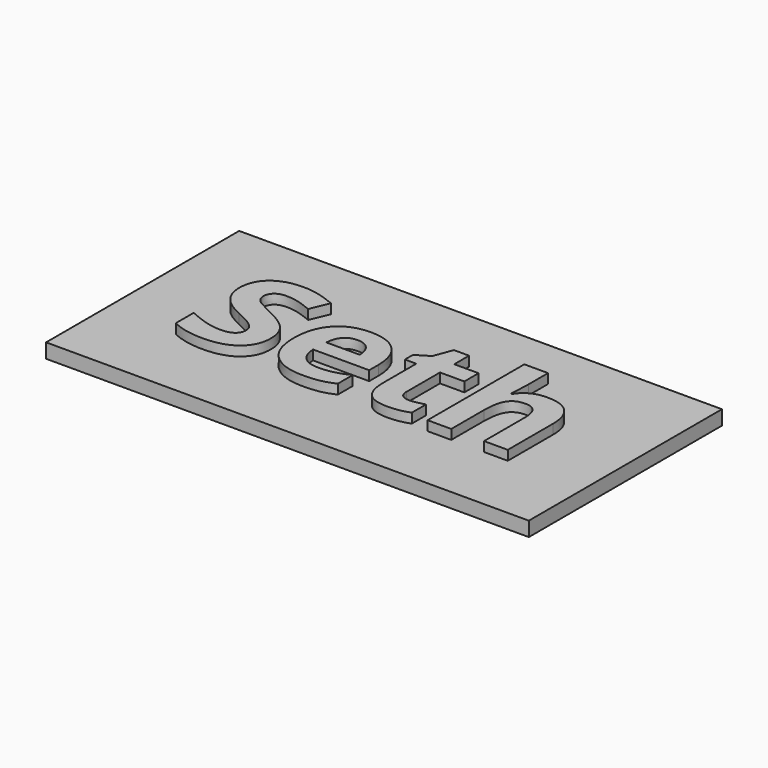
from build123d import *

# Parameters (mm, degrees)
F0_W         = 100
F0_H         = 50
F1_DEPTH     = 3
F2_TEXT_SIZE = 32.9840178084
F3_DEPTH     = 2


# Not quite as in the source:
# - Text() gives the source's letters only with a copy of the font that has no kerning and outlines rounded to 1/6400 em; it was checked with that copy


with BuildPart() as f1:
    # F0 (on Top) → F1 (new body)
    with BuildSketch(Plane.XY):
        with Locations((-50, 25)):
            Rectangle(F0_W, F0_H)
    extrude(amount=F1_DEPTH)

    # F2 (on face) → F3 (join)
    with BuildSketch(Plane.XY.offset(3)):
        with Locations((-86.9271047413, 14.2490956932)):
            Text('Seth', F2_TEXT_SIZE, font='Open Sans', font_style=FontStyle.BOLD, text_align=(TextAlign.LEFT, TextAlign.BOTTOM))
    extrude(amount=F3_DEPTH)


solid = f1.part
